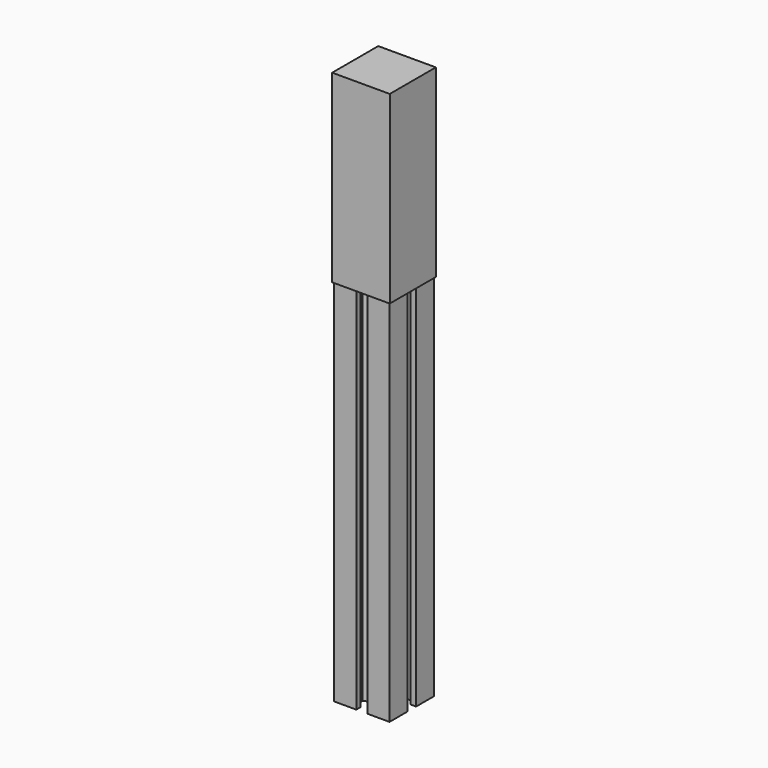
from build123d import *

# Parameters (mm, degrees)
F1_DEPTH = 75
F2_W     = 15.6
F2_H     = 15.6
F3_DEPTH = 50


# Not quite as in the source:
# - ends of sketch curves that miss each other by under 0.0002 mm in the source are joined


with BuildPart() as f1:
    # F0 (on Top) → F1 (new body, symmetric)
    with BuildSketch(Plane.XY):
        Polygon((7.5, 1.5), (7.5, 7.5), (1.5, 7.5), (1.5, 6), (3, 6), (3, 3.5), (1.1461396934, 2.7563427575), (1.1461396934, 2.42764467), (-1.1461396934, 2.42764467), (-1.1461396934, 2.7563427575), (-3, 3.5), (-3, 6), (-1.5, 6), (-1.5, 7.5), (-7.5, 7.5), (-7.5, 1.5), (-6, 1.5), (-6, 3), (-3.5, 3), (-2.7563427575, 1.1461396934), (-2.42764467, 1.1461396934), (-2.42764467, -1.1461396934), (-2.7563427575, -1.1461396934), (-3.5, -3), (-6, -3), (-6, -1.5), (-7.5, -1.5), (-7.5, -7.5), (-1.5, -7.5), (-1.5, -6), (-3, -6), (-3, -3.5), (-1.1461396934, -2.7563427575), (-1.1461396934, -2.42764467), (1.1461396934, -2.42764467), (1.1461396934, -2.7563427575), (3, -3.5), (3, -6), (1.5, -6), (1.5, -7.5), (7.5, -7.5), (7.5, -1.5), (6, -1.5), (6, -3), (3.5, -3), (2.7563427575, -1.1461396934), (2.42764467, -1.1461396934), (2.42764467, 1.1461396934), (2.7563427575, 1.1461396934), (3.5, 3), (6, 3), (6, 1.5), align=None)
    extrude(amount=F1_DEPTH, both=True)

    # F2 (on face) → F3 (join)
    with BuildSketch(Plane.XY.offset(75)):
        Rectangle(F2_W, F2_H)
        Polygon((7.5, 7.5), (7.5, 1.5), (6, 1.5), (6, 3), (3.5, 3), (2.7563427575, 1.1461396934), (2.42764467, 1.1461396934), (2.42764467, -1.1461396934), (2.7563427575, -1.1461396934), (3.5, -3), (6, -3), (6, -1.5), (7.5, -1.5), (7.5, -7.5), (1.5, -7.5), (1.5, -6), (3, -6), (3, -3.5), (1.1461396934, -2.7563427575), (1.1461396934, -2.42764467), (-1.1461396934, -2.42764467), (-1.1461396934, -2.7563427575), (-3, -3.5), (-3, -6), (-1.5, -6), (-1.5, -7.5), (-7.5, -7.5), (-7.5, -1.5), (-6, -1.5), (-6, -3), (-3.5, -3), (-2.7563427575, -1.1461396934), (-2.42764467, -1.1461396934), (-2.42764467, 1.1461396934), (-2.7563427575, 1.1461396934), (-3.5, 3), (-6, 3), (-6, 1.5), (-7.5, 1.5), (-7.5, 7.5), (-1.5, 7.5), (-1.5, 6), (-3, 6), (-3, 3.5), (-1.1461396934, 2.7563427575), (-1.1461396934, 2.42764467), (1.1461396934, 2.42764467), (1.1461396934, 2.7563427575), (3, 3.5), (3, 6), (1.5, 6), (1.5, 7.5), align=None, mode=Mode.SUBTRACT)
    extrude(amount=-F3_DEPTH)


solid = f1.part
